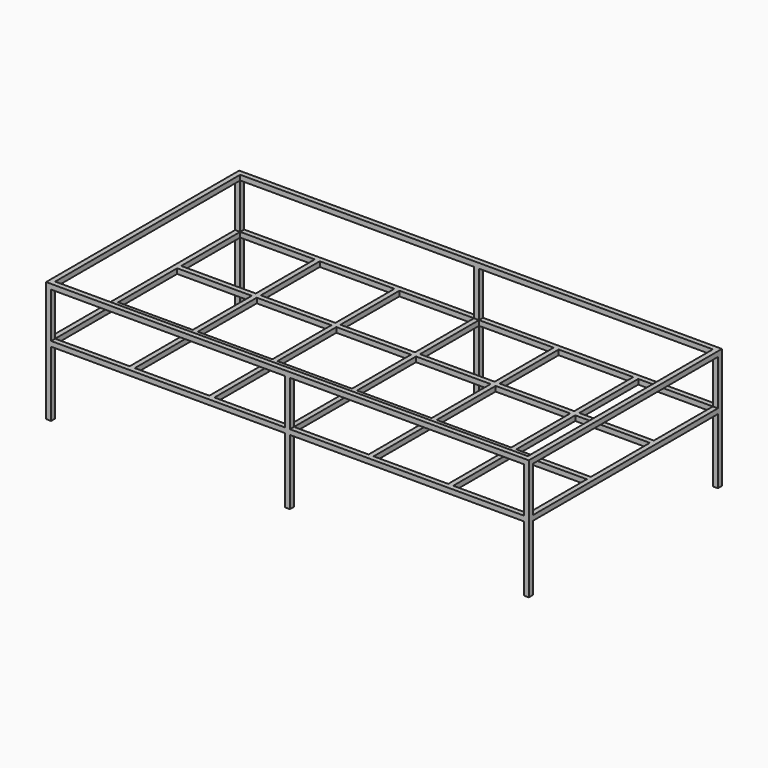
from build123d import *

# Parameters (mm, degrees)
F0_W     = 25.4
F0_H     = 25.4
F0_W_2   = 376.7666666667
F0_H_2   = 372.5333333333
F1_DEPTH = 25.4
F2_DEPTH = 330.2
F3_DEPTH = 254
F4_W     = 2438.4
F4_H     = 1219.2
F4_W_2   = 2387.6
F4_H_2   = 1168.4
F5_DEPTH = 25.4


with BuildPart() as f1:
    # F0 (on Top) → F1 (new body)
    with BuildSketch(Plane.XY):
        with Locations((931.7122847671, -102.1590246889)):
            Rectangle(F0_W, F0_H)
        Polygon((919.0122847671, 1104.3409753111), (-262.0877152329, 1104.3409753111), (-262.0877152329, 1078.9409753111), (-287.4877152329, 1078.9409753111), (-287.4877152329, -89.4590246889), (-262.0877152329, -89.4590246889), (-262.0877152329, -114.8590246889), (919.0122847671, -114.8590246889), (919.0122847671, -89.4590246889), (944.4122847671, -89.4590246889), (944.4122847671, -114.8590246889), (2125.5122847671, -114.8590246889), (2125.5122847671, -89.4590246889), (2150.9122847671, -89.4590246889), (2150.9122847671, 1078.9409753111), (2125.5122847671, 1078.9409753111), (2125.5122847671, 1104.3409753111), (944.4122847671, 1104.3409753111), (944.4122847671, 1078.9409753111), (919.0122847671, 1078.9409753111), align=None)
        with Locations((-73.7043818996, 96.8076419778)):
            Rectangle(F0_W_2, F0_H_2, mode=Mode.SUBTRACT)
        with Locations((328.4622847671, 96.8076419778)):
            Rectangle(F0_W_2, F0_H_2, mode=Mode.SUBTRACT)
        with Locations((730.6289514337, 96.8076419778)):
            Rectangle(F0_W_2, F0_H_2, mode=Mode.SUBTRACT)
        with Locations((-73.7043818996, 494.7409753111)):
            Rectangle(F0_W_2, F0_H_2, mode=Mode.SUBTRACT)
        with Locations((1132.7956181004, 96.8076419778)):
            Rectangle(F0_W_2, F0_H_2, mode=Mode.SUBTRACT)
        with Locations((1534.9622847671, 96.8076419778)):
            Rectangle(F0_W_2, F0_H_2, mode=Mode.SUBTRACT)
        with Locations((1937.1289514337, 96.8076419778)):
            Rectangle(F0_W_2, F0_H_2, mode=Mode.SUBTRACT)
        with Locations((1534.9622847671, 494.7409753111)):
            Rectangle(F0_W_2, F0_H_2, mode=Mode.SUBTRACT)
        with Locations((1937.1289514337, 494.7409753111)):
            Rectangle(F0_W_2, F0_H_2, mode=Mode.SUBTRACT)
        with Locations((328.4622847671, 494.7409753111)):
            Rectangle(F0_W_2, F0_H_2, mode=Mode.SUBTRACT)
        with Locations((730.6289514337, 494.7409753111)):
            Rectangle(F0_W_2, F0_H_2, mode=Mode.SUBTRACT)
        with Locations((-73.7043818996, 892.6743086444)):
            Rectangle(F0_W_2, F0_H_2, mode=Mode.SUBTRACT)
        with Locations((328.4622847671, 892.6743086444)):
            Rectangle(F0_W_2, F0_H_2, mode=Mode.SUBTRACT)
        with Locations((730.6289514337, 892.6743086444)):
            Rectangle(F0_W_2, F0_H_2, mode=Mode.SUBTRACT)
        with Locations((1132.7956181004, 494.7409753111)):
            Rectangle(F0_W_2, F0_H_2, mode=Mode.SUBTRACT)
        with Locations((1132.7956181004, 892.6743086444)):
            Rectangle(F0_W_2, F0_H_2, mode=Mode.SUBTRACT)
        with Locations((1534.9622847671, 892.6743086444)):
            Rectangle(F0_W_2, F0_H_2, mode=Mode.SUBTRACT)
        with Locations((1937.1289514337, 892.6743086444)):
            Rectangle(F0_W_2, F0_H_2, mode=Mode.SUBTRACT)
        with Locations((-274.7877152329, -102.1590246889)):
            Rectangle(F0_W, F0_H)
        with Locations((931.7122847671, 1091.6409753111)):
            Rectangle(F0_W, F0_H)
        with Locations((-274.7877152329, 1091.6409753111)):
            Rectangle(F0_W, F0_H)
        with Locations((2138.2122847671, -102.1590246889)):
            Rectangle(F0_W, F0_H)
        with Locations((2138.2122847671, 1091.6409753111)):
            Rectangle(F0_W, F0_H)
    extrude(amount=F1_DEPTH)

    # F0 (on Top) → F2 (join)
    with BuildSketch(Plane.XY):
        with Locations((-274.7877152329, 1091.6409753111)):
            Rectangle(F0_W, F0_H)
        with Locations((-274.7877152329, -102.1590246889)):
            Rectangle(F0_W, F0_H)
        with Locations((931.7122847671, -102.1590246889)):
            Rectangle(F0_W, F0_H)
        with Locations((2138.2122847671, -102.1590246889)):
            Rectangle(F0_W, F0_H)
        with Locations((2138.2122847671, 1091.6409753111)):
            Rectangle(F0_W, F0_H)
        with Locations((931.7122847671, 1091.6409753111)):
            Rectangle(F0_W, F0_H)
    extrude(amount=-F2_DEPTH)

    # F0 (on Top) → F3 (join)
    with BuildSketch(Plane.XY):
        with Locations((-274.7877152329, 1091.6409753111)):
            Rectangle(F0_W, F0_H)
        with Locations((931.7122847671, 1091.6409753111)):
            Rectangle(F0_W, F0_H)
        with Locations((-274.7877152329, -102.1590246889)):
            Rectangle(F0_W, F0_H)
        with Locations((931.7122847671, -102.1590246889)):
            Rectangle(F0_W, F0_H)
        with Locations((2138.2122847671, -102.1590246889)):
            Rectangle(F0_W, F0_H)
        with Locations((2138.2122847671, 1091.6409753111)):
            Rectangle(F0_W, F0_H)
    extrude(amount=F3_DEPTH)

    # F4 (on face) → F5 (join)
    with BuildSketch(Plane.XY.offset(254)):
        with Locations((931.7122847671, 494.7409753111)):
            Rectangle(F4_W, F4_H)
        with Locations((931.7122847671, 494.7409753111)):
            Rectangle(F4_W_2, F4_H_2, mode=Mode.SUBTRACT)
    extrude(amount=F5_DEPTH)


solid = f1.part
